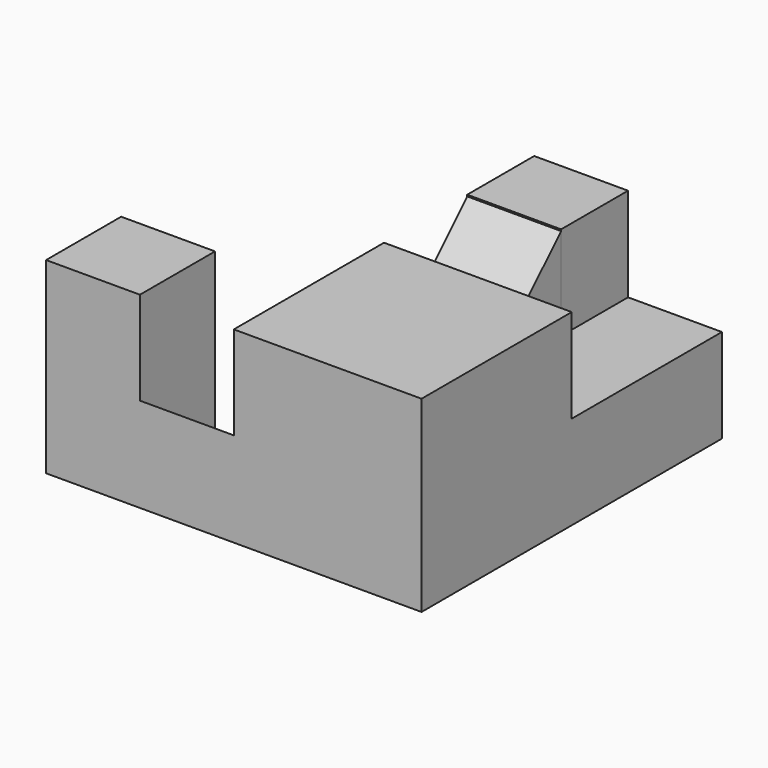
from build123d import *

# Parameters (mm, degrees)
F0_W        = 8
F0_H        = 8
F1_DEPTH    = 8.05
F2_DEPTH    = 16
F3_SIZE     = 7.99999
F4_DEPTH    = 16
F5_DEPTH    = 8
F0_H_2      = 7.1334964926
F6_DEPTH    = 16
F0_H_3      = 8.8665035074
F7_DEPTH    = 16
F8_T1_DEPTH = 54.2902937834


# Not quite as in the source:
# - a fillet or chamfer that OpenCascade refuses, or shapes differently, is made with other operations: its cross-section is extruded or revolved along the edge and cut away or added
# - a fillet or chamfer is up to 0.001 mm smaller than in the source, because OpenCascade refuses the exact size


with BuildPart() as f1:
    # F0 (on Top) → F1 (new body)
    with BuildSketch(Plane.XY):
        with Locations((-35.1440954627, 9.3118814863)):
            Rectangle(F0_W, F0_H)
    extrude(amount=F1_DEPTH)

    # F0 (on Top) → F2 (join)
    with BuildSketch(Plane.XY):
        Polygon((-23.1440954627, 21.3118814863), (-31.1440954627, 21.3118814863), (-31.1440954627, 13.3118814863), (-31.1440954627, 5.3118814863), (-15.1440954627, 5.3118814863), (-15.1440954627, 21.3118814863), align=None)
    extrude(amount=F2_DEPTH)

    # F3 (size 8 in the source; OpenCascade refuses exactly that, so slightly less here)
    f3_edges = [f1.edges().sort_by_distance(p)[0] for p in [
        (-35.144095, 13.311881, 8.05),
    ]]
    chamfer(f3_edges, length=F3_SIZE)

    # F0 (on Top) → F4 (join)
    with BuildSketch(Plane.XY):
        with Locations((-43.1440954627, 9.3118814863)):
            Rectangle(F0_W, F0_H)
    extrude(amount=F4_DEPTH)

    # F0 (on Top) → F5 (join)
    with BuildSketch(Plane.XY):
        Polygon((-15.1440954627, 37.3118814863), (-23.1440954627, 37.3118814863), (-23.1440954627, 30.1783849937), (-23.1440954627, 21.3118814863), (-15.1440954627, 21.3118814863), align=None)
    extrude(amount=F5_DEPTH)

    # F0 (on Top) → F6 (join)
    with BuildSketch(Plane.XY):
        with Locations((-27.1440954627, 33.74513324)):
            Rectangle(F0_W, F0_H_2)
    extrude(amount=F6_DEPTH)


with BuildPart() as f7:
    # F0 (on Top) → F7 (new body)
    with BuildSketch(Plane.XY):
        with Locations((-27.1440954627, 25.74513324)):
            Rectangle(F0_W, F0_H_3)
    extrude(amount=F7_DEPTH)

    # F8: chamfer of 9 on 1 edges, made by hand

    # F8_s2 → F8_t1 (cut)
    with BuildSketch(Plane.YZ.offset(-54.2892423544)):
        Polygon((21.3118814863, 7), (30.3118814863, 16), (21.3118814863, 16), align=None)
    extrude(amount=F8_T1_DEPTH, mode=Mode.SUBTRACT)


solid = Compound([f1.part, f7.part])
